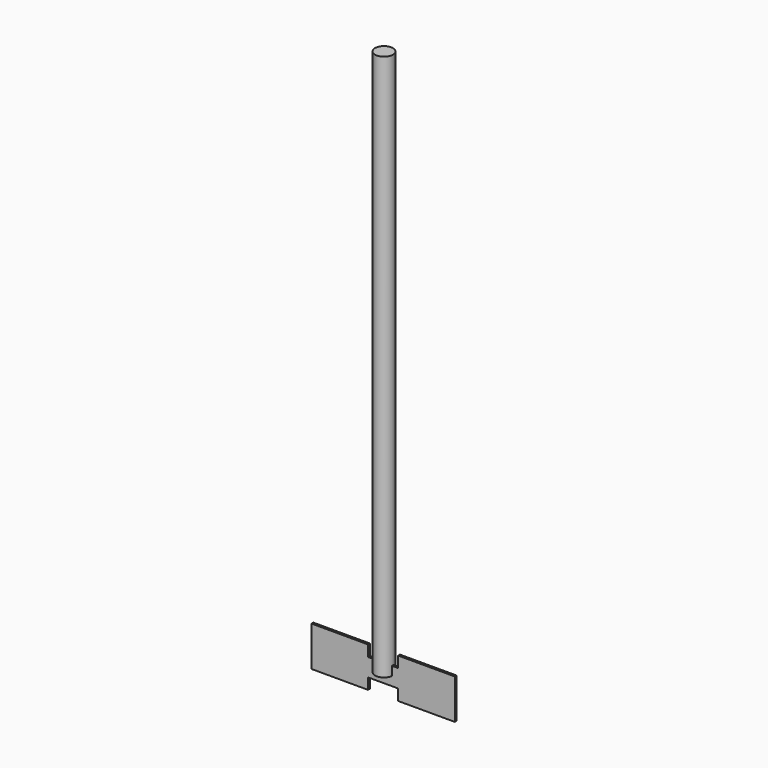
from build123d import *

# Parameters (mm, degrees)
F0_W     = 85.7623966645
F0_H     = 50.8
F2_DEPTH = 3.175
F1_R     = 25.4
F4_DEPTH = 1549.4


# Not quite as in the source:
# - the program builds the solid bodies; features that only make, move or delete a surface that nothing else refers to are left out


with BuildPart() as f2:
    # F0 (on Front) → F2 (new body, symmetric)
    with BuildSketch(Plane.XZ):
        Rectangle(F0_W, F0_H)
        Polygon((42.8811983322, 56.6644097805), (42.8811983322, 25.4), (42.8811983322, -25.4), (42.8811983322, -56.6644097805), (203.2, -56.6644097805), (203.2, 56.6644097805), align=None)
        Polygon((-42.8811983322, -25.4), (-42.8811983322, 25.4), (-42.8811983322, 56.6644097805), (-203.2, 56.6644097805), (-203.2, -56.6644097805), (-42.8811983322, -56.6644097805), align=None)
    extrude(amount=F2_DEPTH, both=True)

    # F1 (on Top) → F4 (join)
    with BuildSketch(Plane.XY):
        Circle(F1_R)
    extrude(amount=F4_DEPTH)


solid = f2.part
